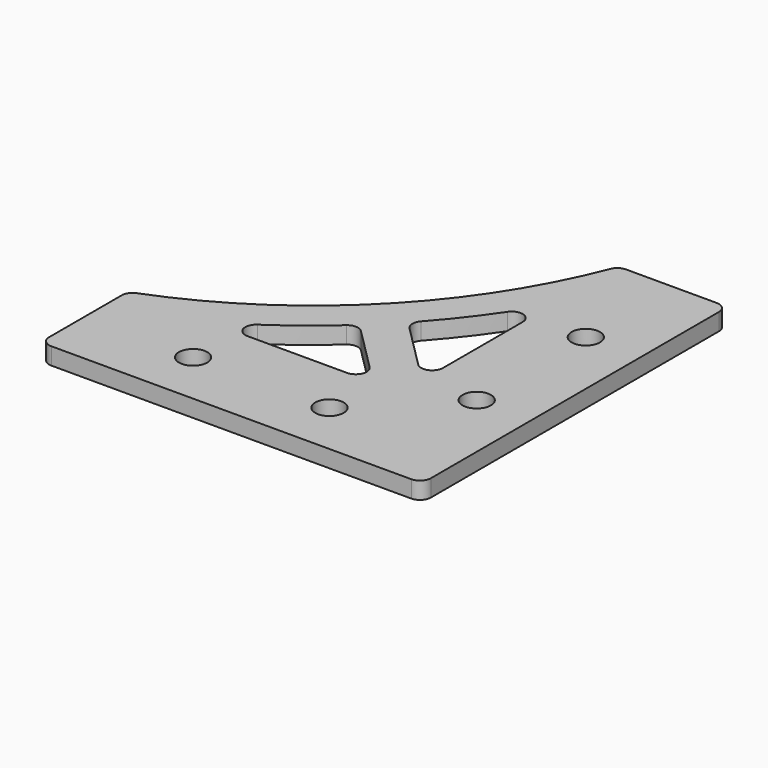
from build123d import *

# Parameters (mm, degrees)
F1_DEPTH  = 3.125
F2_W      = 6
F2_H      = 50
F2_W_2    = 50
F2_H_2    = 6
F3_DEPTH  = 2
F4_R      = 2.6
F5_DEPTH  = 25
F6_W      = 6
F6_H      = 12.6
F6_H_2    = 15.2
F7_DEPTH  = 2
F8_W      = 12.6
F8_H      = 6
F8_W_2    = 15.2
F9_DEPTH  = 2
F10_R     = 2
F12_DEPTH = 25
F13_R     = 2


# Not quite as in the source:
# - a feature names something its author has since deleted; it is built from what else it names


with BuildPart() as f1:
    # F0 (on Top) → F1 (new body)
    with BuildSketch(Plane.XY):
        with BuildLine():
            Line((35, 35), (15, 35))
            ThreePointArc((15, 35), (-4.5539513718, 4.5539513718), (-35, -15))
            Line((-35, -15), (-35, -35))
            Line((-35, -35), (35, -35))
            Line((35, -35), (35, 35))
        make_face()
    extrude(amount=F1_DEPTH)

    # F2 (on face) → F3 (join)
    with BuildSketch(Plane(origin=(0, 0, 0), x_dir=(1, 0, 0), z_dir=(0, 0, -1))):
        with Locations((25, -10)):
            Rectangle(F2_W, F2_H)
        with Locations((-10, 25)):
            Rectangle(F2_W_2, F2_H_2)
    extrude(amount=F3_DEPTH)

    # F4 (on face) → F5 (cut)
    with BuildSketch(Plane(origin=(0, 0, -2), x_dir=(1, 0, 0), z_dir=(0, 0, -1))):
        with Locations((25, -15)):
            Circle(F4_R)
        with Locations((25, 10)):
            Circle(F4_R)
        with Locations((10, 25)):
            Circle(F4_R)
        with Locations((-15, 25)):
            Circle(F4_R)
    extrude(amount=-F5_DEPTH, mode=Mode.SUBTRACT)

    # F6 (on face) → F7 (cut)
    with BuildSketch(Plane(origin=(0, 0, -2), x_dir=(1, 0, 0), z_dir=(0, 0, -1))):
        with Locations((25, 8.7)):
            Rectangle(F6_W, F6_H)
        with Locations((25, -15)):
            Rectangle(F6_W, F6_H_2)
    extrude(amount=-F7_DEPTH, mode=Mode.SUBTRACT)

    # F8 (on face) → F9 (cut)
    with BuildSketch(Plane(origin=(0, 0, -2), x_dir=(1, 0, 0), z_dir=(0, 0, -1))):
        with Locations((8.7, 25)):
            Rectangle(F8_W, F8_H)
        with Locations((-15, 25)):
            Rectangle(F8_W_2, F8_H)
    extrude(amount=-F9_DEPTH, mode=Mode.SUBTRACT)

    # F10
    f10_edges = [f1.edges().sort_by_distance(p)[0] for p in [
        (35, 35, 1.5625),
        (15, 35, 1.5625),
        (-35, -15, 1.5625),
        (-35, -35, 1.5625),
        (35, -35, 1.5625),
    ]]
    fillet(f10_edges, radius=F10_R)

    # F11 (on Top) → F12 (cut)
    with BuildSketch(Plane.XY):
        with BuildLine():
            Line((15, -10.0502525317), (15, 20))
            ThreePointArc((15, 20), (9.1151461726, 10.9887424757), (2.2488038315, 2.7009436368))
            Line((2.2488038315, 2.7009436368), (15, -10.0502525317))
        make_face()
        with BuildLine():
            ThreePointArc((-2.7009436368, -2.2488038315), (-10.9887424757, -9.1151461726), (-20, -15))
            Line((-20, -15), (10.0502525317, -15))
            Line((10.0502525317, -15), (-2.7009436368, -2.2488038315))
        make_face()
    extrude(amount=F12_DEPTH, mode=Mode.SUBTRACT)

    # F13
    f13_edges = [f1.edges().sort_by_distance(p)[0] for p in [
        (15, 20, 1.5625),
        (-20, -15, 1.5625),
        (2.248804, 2.700944, 1.5625),
        (-2.700944, -2.248804, 1.5625),
        (10.050253, -15, 1.5625),
        (15, -10.050253, 1.5625),
    ]]
    fillet(f13_edges, radius=F13_R)


solid = f1.part
